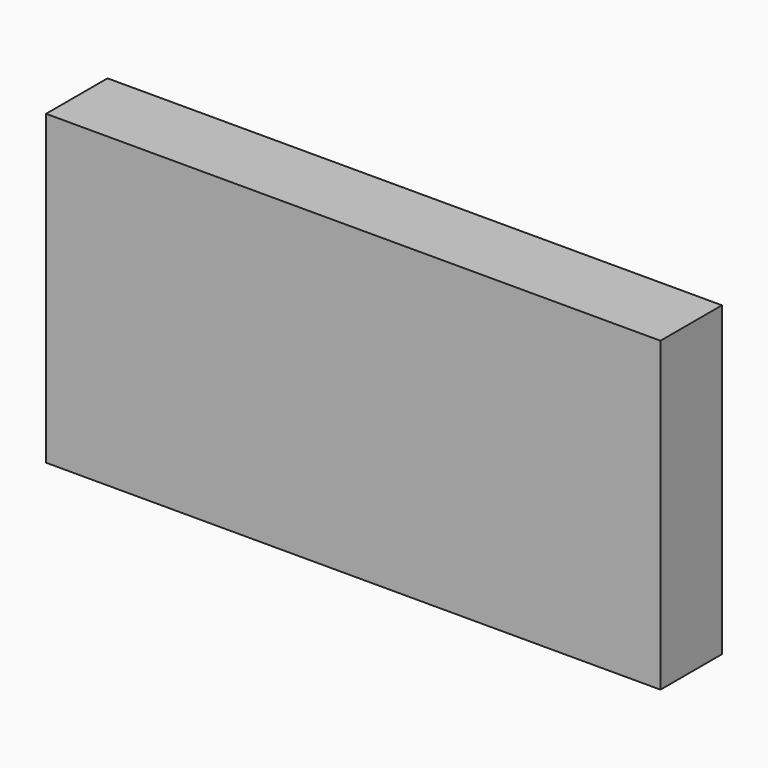
from build123d import *

# Parameters (mm, degrees)
F0_W     = 80
F0_H     = 40
F1_DEPTH = 10


# Not quite as in the source:
# - the program builds the solid bodies; features that only make, move or delete a surface that nothing else refers to are left out


with BuildPart() as f1:
    # F0 (on Front) → F1 (new body)
    with BuildSketch(Plane.XZ):
        Rectangle(F0_W, F0_H)
    extrude(amount=F1_DEPTH)


solid = f1.part
